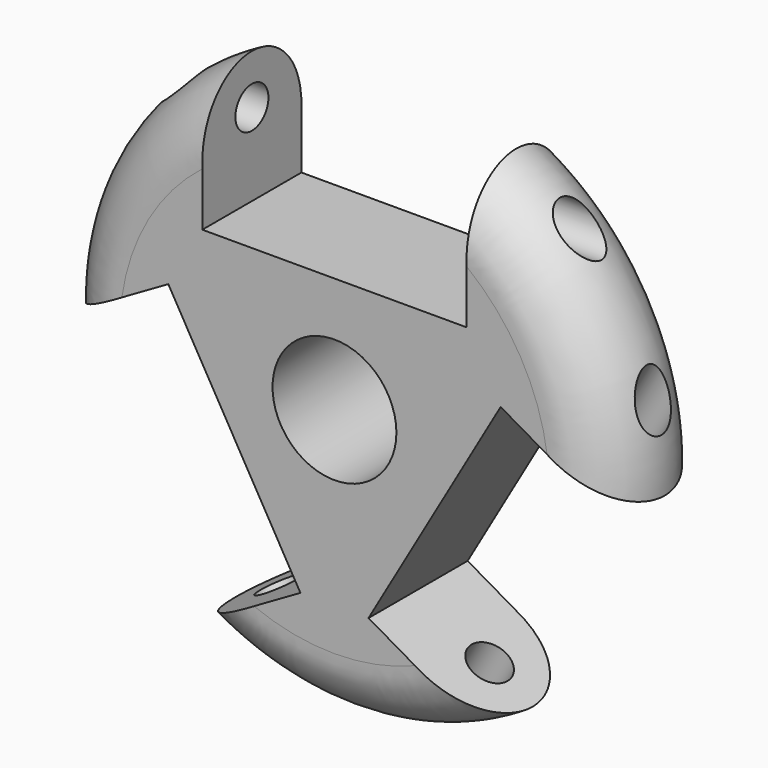
from build123d import *

# Parameters (mm, degrees)
F2_R            = 4.7625
F2_W            = 20.32
F2_H            = 25.4
F3_DEPTH        = 4.773421975
F3_DEPTH_BACK   = 4.773421975
F4_R            = 1.5875
F5_DEPTH        = 21.5910001
F5_DEPTH_BACK   = 21.5910001
F5_COPIES_COUNT = 3


# Not quite as in the source:
# - a pattern or mirror of a feature is missing from the dataset's text; its kind, count and spacing are read off the source's solid


with BuildPart() as f1:
    # F0 (on Right) → F1 (revolve)
    with BuildSketch(Plane.YZ):
        with BuildLine():
            Line((-4.7625, 0), (0, 0))
            Line((0, 0), (4.7625, 0))
            Line((4.7625, 0), (4.7625, 16.51))
            ThreePointArc((4.7625, 16.51), (0, 21.59), (-4.7625, 16.51))
            Line((-4.7625, 16.51), (-4.7625, 0))
        make_face()
    revolve(axis=Axis((0, -2.38125, 0), (0, -1, 0)))

    # F2 (on Front) → F3 (cut, two sides)
    with BuildSketch(Plane.XZ) as f3_sk:
        Circle(F2_R)
        with Locations((0, 21.59)):
            Rectangle(F2_W, F2_H)
        Polygon((-12.7789658396, 4.3538181024), (-34.7760110958, -8.3461818976), (-24.6160110958, -25.9438181024), (-2.6189658396, -13.2438181024), align=None)
        Polygon((2.6189658396, -13.2438181024), (24.6160110958, -25.9438181024), (34.7760110958, -8.3461818976), (12.7789658396, 4.3538181024), align=None)
    extrude(amount=-F3_DEPTH, mode=Mode.SUBTRACT)
    extrude(f3_sk.sketch, amount=F3_DEPTH_BACK, mode=Mode.SUBTRACT)

    # F4 (on Right) → F5 (cut, two sides)
    with BuildSketch(Plane.YZ) as f5_sk:
        with Locations((0, 15.24)):
            Circle(F4_R)
    f5 = extrude(amount=-F5_DEPTH, mode=Mode.SUBTRACT) + extrude(f5_sk.sketch, amount=F5_DEPTH_BACK, mode=Mode.SUBTRACT)

    # F5_copies: F5 ×3 about axis
    f5_copies_axis = Axis((0, 0, 0), (0, 1, 0))
    for i in range(1, F5_COPIES_COUNT):
        add(f5.rotate(f5_copies_axis, i * 360 / F5_COPIES_COUNT), mode=Mode.SUBTRACT)


solid = f1.part
